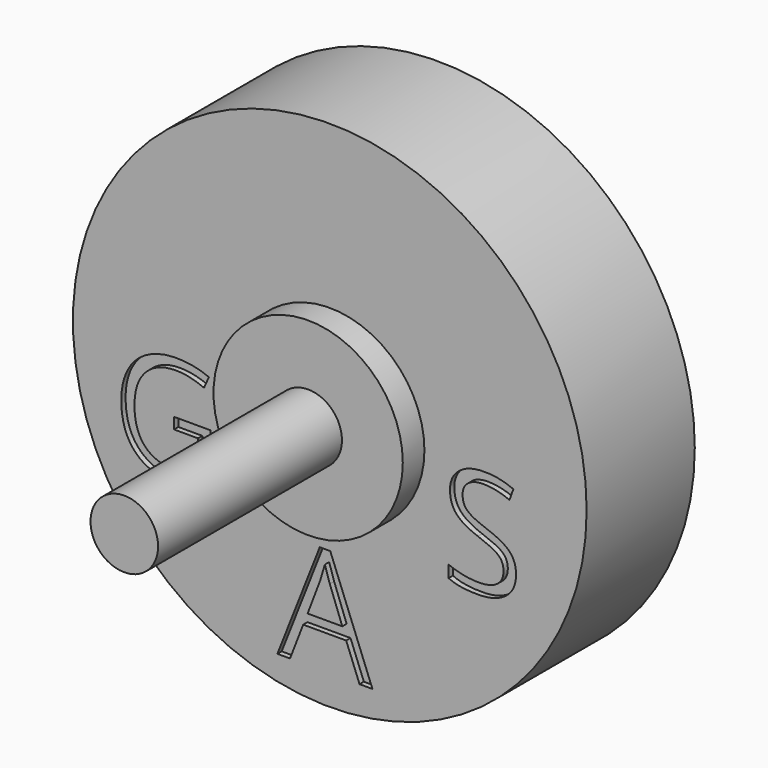
from build123d import *

# Parameters (mm, degrees)
F0_R         = 12.5
F1_DEPTH     = 145
F0_R_2       = 95
F0_R_3       = 35
F2_DEPTH     = 50
F3_DEPTH     = 60
F4_TEXT_SIZE = 55.5555555556
F5_DEPTH     = 2


# Not quite as in the source:
# - Text() gives the source's letters only with a copy of the font that has no kerning and outlines rounded to 1/6400 em; it was checked with that copy


with BuildPart() as f1:
    # F0 (on Front) → F1 (new body)
    with BuildSketch(Plane.XZ):
        Circle(F0_R)
    extrude(amount=F1_DEPTH)



with BuildPart() as f2:
    # F0 (on Front) → F2 (new body)
    with BuildSketch(Plane.XZ):
        Circle(F0_R_2)
        Circle(F0_R_3, mode=Mode.SUBTRACT)
    extrude(amount=F2_DEPTH)


with BuildPart() as f1_1:
    add(f1.part)

    add(f2.part)  # F3 merges F2
    # F0 (on Front) → F3 (join)
    with BuildSketch(Plane.XZ):
        Circle(F0_R_3)
        Circle(F0_R, mode=Mode.SUBTRACT)
    extrude(amount=F3_DEPTH)

    # F4 (on face) → F5 (cut)
    with BuildSketch(Plane.XZ.offset(50)):
        with Locations((-80.5048076169, -40)):
            Text('G', F4_TEXT_SIZE, font='Open Sans', text_align=(TextAlign.LEFT, TextAlign.BOTTOM))
        with Locations((-19.3793402778, -83.9627224204)):
            Text('A', F4_TEXT_SIZE, font='Open Sans', text_align=(TextAlign.LEFT, TextAlign.BOTTOM))
        with Locations((41.0689688897, -40)):
            Text('S', F4_TEXT_SIZE, font='Open Sans', text_align=(TextAlign.LEFT, TextAlign.BOTTOM))
    extrude(amount=-F5_DEPTH, mode=Mode.SUBTRACT)


solid = f1_1.part
